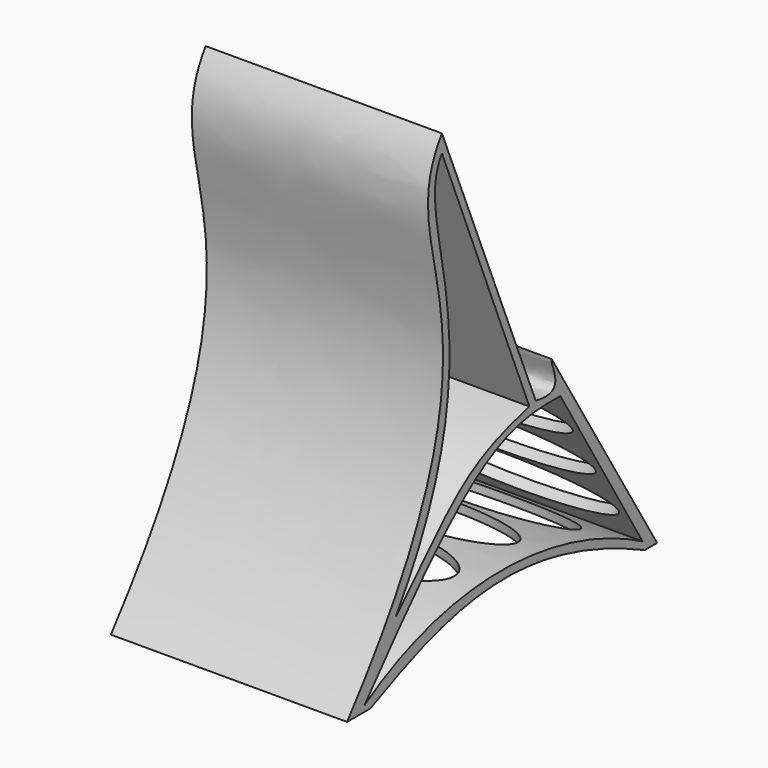
from build123d import *

# Parameters (mm, degrees)
F1_DEPTH  = 70
F5_DEPTH  = 295
F7_DEPTH  = 295
F9_REACH  = 142.245355745
F11_REACH = 198.6043545962


# Not quite as in the source:
# - an extrude ends at something that could not be found from the text; its depth is read off the source's solid


with BuildPart() as f1:
    # F0 (on Right) → F1 (new body)
    with BuildSketch(Plane.YZ):
        with BuildLine():
            add(Edge.make_bspline(
                [(-65.0536715984, 0), (2.1839654073, 84.6990346909), (-50.6073869765, 110.0246235728), (-29.9188829958, 139.2738819122)],
                knots=[0, 0, 0, 0, 143.6372777278, 143.6372777278, 143.6372777278, 143.6372777278], degree=3))
            Line((-65.0536715984, 0), (-56.4117916499, 0))
            add(Edge.make_bspline(
                [(-56.4117916499, 0), (-27.936052531, 13.126176782), (-1.7122571589, 22.8152908385), (45.2086254954, 0)],
                knots=[0, 0, 0, 0, 101.6204171453, 101.6204171453, 101.6204171453, 101.6204171453], degree=3))
            Line((45.2086254954, 0), (49.8031899333, 0))
            add(Edge.make_bspline(
                [(49.8031899333, 0), (36.7837014298, 21.2773953875), (23.7642129262, 42.554790775), (10.7447244227, 63.8321861625)],
                knots=[0, 0, 0, 0, 74.8338941812, 74.8338941812, 74.8338941812, 74.8338941812], degree=3))
            add(Edge.make_bspline(
                [(4.8285723044, 55.386091928), (17.0853175535, 52.8970839186), (9.9300900474, 62.5007674098), (10.7447244227, 63.8321861625)],
                knots=[0, 0, 0, 0, 10.3120009554, 10.3120009554, 10.3120009554, 10.3120009554], degree=3))
            Line((4.8285723044, 55.386091928), (-29.9188829958, 139.2738819122))
        make_face()
        with BuildLine():
            add(Edge.make_bspline(
                [(-58.5831403732, 1.7520016991), (-26.5599957202, 21.9477838837), (12.6107810065, 19.9717469513), (44.4163493812, 2.5945331436)],
                knots=[0, 0, 0, 0, 103.0029356325, 103.0029356325, 103.0029356325, 103.0029356325], degree=3))
            add(Edge.make_bspline(
                [(-58.5831403732, 1.7520016991), (-21.4064326137, 45.8795949817), (-9.4003584236, 53.8836456835), (13.9829870313, 52.8689771891)],
                knots=[0, 0, 0, 0, 88.7625373102, 88.7625373102, 88.7625373102, 88.7625373102], degree=3))
            Line((13.9829870313, 52.8689771891), (44.4163493812, 2.5945331436))
        make_face(mode=Mode.SUBTRACT)
        with BuildLine():
            Line((-29.9037508667, 134.0290158987), (2.4867416879, 54.8259804102))
            add(Edge.make_bspline(
                [(-47.1550263464, 19.8711045086), (-25.1918910405, 42.0185283913), (-22.0024906202, 48.7895191963), (2.4867416879, 54.8259804102)],
                knots=[0, 0, 0, 0, 61.0628862948, 61.0628862948, 61.0628862948, 61.0628862948], degree=3))
            add(Edge.make_bspline(
                [(-47.1550263464, 19.8711045086), (-6.9014942273, 80.1363065839), (-41.790433228, 117.2437295318), (-29.9037508667, 134.0290158987)],
                knots=[0, 0, 0, 0, 115.4540395076, 115.4540395076, 115.4540395076, 115.4540395076], degree=3))
        make_face(mode=Mode.SUBTRACT)
    extrude(amount=F1_DEPTH)

    # F4 (on face) → F5 (cut, through all)
    with BuildSketch(Plane.XY.offset(139.2738819122)):
        with BuildLine():
            add(Edge.make_bspline(
                [(2.5, -10.4053849354), (2.5, -25.1278167998), (51.25, -17.7666008676), (100, -10.4053849354), (51.25, -3.0441690033), (2.5, 4.3170469289), (2.5, -10.4053849354)],
                knots=[0, 0, 0, 2.0943951024, 2.0943951024, 4.1887902048, 4.1887902048, 6.2831853072, 6.2831853072, 6.2831853072], degree=2, weights=[1, 0.5, 1, 0.5, 1, 0.5, 1]))
        make_face()
        with BuildLine():
            add(Edge.make_bspline(
                [(2.5, 7.5946150646), (2.5, -7.1278167998), (51.25, 0.2333991324), (100, 7.5946150646), (51.25, 14.9558309967), (2.5, 22.3170469289), (2.5, 7.5946150646)],
                knots=[0, 0, 0, 2.0943951024, 2.0943951024, 4.1887902048, 4.1887902048, 6.2831853072, 6.2831853072, 6.2831853072], degree=2, weights=[1, 0.5, 1, 0.5, 1, 0.5, 1]))
        make_face()
        with BuildLine():
            add(Edge.make_bspline(
                [(2.5, 25.5946150646), (2.5, 10.8721832002), (51.25, 18.2333991324), (100, 25.5946150646), (51.25, 32.9558309967), (2.5, 40.3170469289), (2.5, 25.5946150646)],
                knots=[0, 0, 0, 2.0943951024, 2.0943951024, 4.1887902048, 4.1887902048, 6.2831853072, 6.2831853072, 6.2831853072], degree=2, weights=[1, 0.5, 1, 0.5, 1, 0.5, 1]))
        make_face()
        with BuildLine():
            add(Edge.make_bspline(
                [(2.5, 43.5946150646), (2.5, 28.8721832002), (51.25, 36.2333991324), (100, 43.5946150646), (51.25, 50.9558309967), (2.5, 58.3170469289), (2.5, 43.5946150646)],
                knots=[0, 0, 0, 2.0943951024, 2.0943951024, 4.1887902048, 4.1887902048, 6.2831853072, 6.2831853072, 6.2831853072], degree=2, weights=[1, 0.5, 1, 0.5, 1, 0.5, 1]))
        make_face()
    extrude(amount=F5_DEPTH, mode=Mode.SUBTRACT)

    # F6 (on face) → F7 (cut, through all)
    with BuildSketch(Plane.XY.offset(139.2738819122)):
        with BuildLine():
            add(Edge.make_bspline(
                [(17.502522096, -29.3557792902), (17.502522096, -36.1721548588), (44.1732993349, -32.7639670745), (70.8440765738, -29.3557792902), (44.1732993349, -25.9475915059), (17.502522096, -22.5394037216), (17.502522096, -29.3557792902)],
                knots=[0, 0, 0, 2.0943951024, 2.0943951024, 4.1887902048, 4.1887902048, 6.2831853072, 6.2831853072, 6.2831853072], degree=2, weights=[1, 0.5, 1, 0.5, 1, 0.5, 1]))
        make_face()
    extrude(amount=F7_DEPTH, mode=Mode.SUBTRACT)

    f9_end = f1.faces().sort_by_distance((35, 30.273957178, 31.9160930812))[0]
    # F8 (on face) → F9 (cut, up to a face of the model that its end follows)
    with BuildSketch(Plane(origin=(0, 33.6545084372, 20.372574365), x_dir=(1, 0, 0), z_dir=(0, -0.8554692211, -0.5178536586))):
        with BuildLine():
            add(Edge.make_bspline(
                [(67.5, 23.4277807176), (67.5, 36.9762650043), (18.75, 30.202022861), (-30, 23.4277807176), (18.75, 16.6535385743), (67.5, 9.8792964309), (67.5, 23.4277807176)],
                knots=[0, 0, 0, 2.0943951024, 2.0943951024, 4.1887902048, 4.1887902048, 6.2831853072, 6.2831853072, 6.2831853072], degree=2, weights=[1, 0.5, 1, 0.5, 1, 0.5, 1]))
        make_face()
        with BuildLine():
            add(Edge.make_bspline(
                [(67.5, 6.9277807176), (67.5, 20.4762650043), (18.75, 13.702022861), (-30, 6.9277807176), (18.75, 0.1535385743), (67.5, -6.6207035691), (67.5, 6.9277807176)],
                knots=[0, 0, 0, 2.0943951024, 2.0943951024, 4.1887902048, 4.1887902048, 6.2831853072, 6.2831853072, 6.2831853072], degree=2, weights=[1, 0.5, 1, 0.5, 1, 0.5, 1]))
        make_face()
        with BuildLine():
            add(Edge.make_bspline(
                [(67.5, -9.5722192824), (67.5, 3.9762650043), (18.75, -2.797977139), (-30, -9.5722192824), (18.75, -16.3464614257), (67.5, -23.1207035691), (67.5, -9.5722192824)],
                knots=[0, 0, 0, 2.0943951024, 2.0943951024, 4.1887902048, 4.1887902048, 6.2831853072, 6.2831853072, 6.2831853072], degree=2, weights=[1, 0.5, 1, 0.5, 1, 0.5, 1]))
        make_face()
    f9_long = extrude(amount=-F9_REACH, mode=Mode.PRIVATE)
    add(split(f9_long, bisect_by=f9_end, keep=Keep.BOTTOM, mode=Mode.PRIVATE), mode=Mode.SUBTRACT)

    f11_end = f1.faces().sort_by_distance((35, -7.0018043916, 16.2631409185))[0]
    # F10 (on Top) → F11 (cut, up to a face of the model that its end follows)
    with BuildSketch(Plane.XY):
        with BuildLine():
            add(Edge.make_bspline(
                [(62.8528258204, -38.5428890586), (62.8528258204, -20.8609774983), (21.0735870898, -29.7019332784), (-20.7056516409, -38.5428890586), (21.0735870898, -47.3838448388), (62.8528258204, -56.2248006189), (62.8528258204, -38.5428890586)],
                knots=[0, 0, 0, 2.0943951024, 2.0943951024, 4.1887902048, 4.1887902048, 6.2831853072, 6.2831853072, 6.2831853072], degree=2, weights=[1, 0.5, 1, 0.5, 1, 0.5, 1]))
        make_face()
        with BuildLine():
            add(Edge.make_bspline(
                [(62.8528258204, -15.9428890586), (62.8528258204, 1.7390225017), (21.0735870898, -7.1019332784), (-20.7056516409, -15.9428890586), (21.0735870898, -24.7838448388), (62.8528258204, -33.6248006189), (62.8528258204, -15.9428890586)],
                knots=[0, 0, 0, 2.0943951024, 2.0943951024, 4.1887902048, 4.1887902048, 6.2831853072, 6.2831853072, 6.2831853072], degree=2, weights=[1, 0.5, 1, 0.5, 1, 0.5, 1]))
        make_face()
        with BuildLine():
            add(Edge.make_bspline(
                [(62.8528258204, 6.6571109414), (62.8528258204, 24.3390225017), (21.0735870898, 15.4980667216), (-20.7056516409, 6.6571109414), (21.0735870898, -2.1838448388), (62.8528258204, -11.0248006189), (62.8528258204, 6.6571109414)],
                knots=[0, 0, 0, 2.0943951024, 2.0943951024, 4.1887902048, 4.1887902048, 6.2831853072, 6.2831853072, 6.2831853072], degree=2, weights=[1, 0.5, 1, 0.5, 1, 0.5, 1]))
        make_face()
        with BuildLine():
            add(Edge.make_bspline(
                [(62.8528258204, 29.2571109414), (62.8528258204, 46.9390225017), (21.0735870898, 38.0980667216), (-20.7056516409, 29.2571109414), (21.0735870898, 20.4161551612), (62.8528258204, 11.5751993811), (62.8528258204, 29.2571109414)],
                knots=[0, 0, 0, 2.0943951024, 2.0943951024, 4.1887902048, 4.1887902048, 6.2831853072, 6.2831853072, 6.2831853072], degree=2, weights=[1, 0.5, 1, 0.5, 1, 0.5, 1]))
        make_face()
    f11_long = extrude(amount=F11_REACH, mode=Mode.PRIVATE)
    add(split(f11_long, bisect_by=f11_end, keep=Keep.BOTTOM, mode=Mode.PRIVATE), mode=Mode.SUBTRACT)


solid = f1.part
